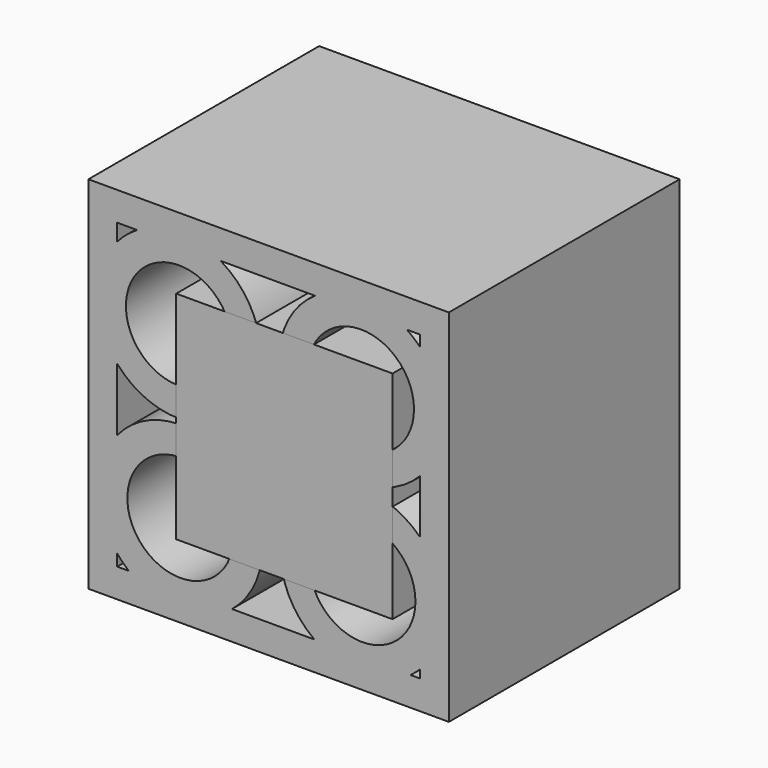
from build123d import *

# Parameters (mm, degrees)
F1_R     = 4.6736
F1_W     = 31.623
F1_H     = 16.891
F2_DEPTH = 25.4
F3_T     = -2.54
F0_W     = 19.05
F0_H     = 19.05
F5_DEPTH = 25.4


# Not quite as in the source:
# - the program builds the solid bodies; features that only make, move or delete a surface that nothing else refers to are left out


with BuildPart() as f2:
    # F1 (on Front) → F2 (new body)
    with BuildSketch(Plane.XZ):
        Polygon((15.875, 1.016), (15.875, 15.875), (-15.875, 15.875), (-15.875, -15.875), (-15.748, -15.875), (-15.748, 1.016), align=None)
        with Locations((-7.8961248569, 7.1288868002)):
            Circle(F1_R, mode=Mode.SUBTRACT)
        with Locations((8.128, 7.366)):
            Circle(F1_R, mode=Mode.SUBTRACT)
        with Locations((0.0635, -7.4295)):
            Rectangle(F1_W, F1_H)
        with Locations((-7.7691248569, -7.7301131998)):
            Circle(F1_R, mode=Mode.SUBTRACT)
        with Locations((8.255, -7.493)):
            Circle(F1_R, mode=Mode.SUBTRACT)
    extrude(amount=F2_DEPTH)

    # F3
    f3_openings = [f2.faces().sort_by_distance(p)[0] for p in [
        (-0.06714, -25.4, 0.068119),
    ]]
    offset(amount=F3_T, openings=f3_openings)


with BuildPart() as f5:
    # F0 (on Front) → F5 (new body)
    with BuildSketch(Plane.XZ):
        with Locations((1.3871352458, 0)):
            Rectangle(F0_W, F0_H)
    extrude(amount=F5_DEPTH)


solid = Compound([f2.part, f5.part])
